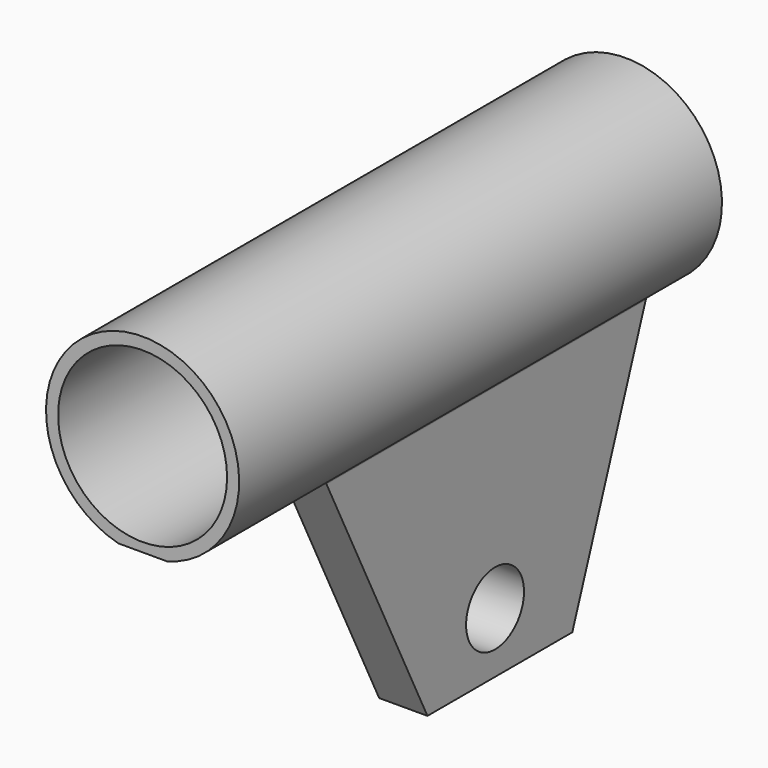
from build123d import *

# Parameters (mm, degrees)
F0_R     = 7
F1_DEPTH = 50
F3_R     = 3
F4_DEPTH = 25
F5_R     = 1.5


with BuildPart() as f1:
    # F0 (on Front) → F1 (new body)
    with BuildSketch(Plane.XZ):
        with BuildLine():
            Line((2, -30), (2, -7.7459666924))
            ThreePointArc((2, -7.7459666924), (0, 8), (-2, -7.7459666924))
            Line((-2, -7.7459666924), (-2, -30))
            Line((-2, -30), (0, -30))
            Line((0, -30), (2, -30))
        make_face()
        Circle(F0_R, mode=Mode.SUBTRACT)
    extrude(amount=F1_DEPTH)

    # F3 (on face) → F4 (cut)
    with BuildSketch(Plane(origin=(-2, 0, 0), x_dir=(0, -1, 0), z_dir=(-1, 0, 0))):
        Polygon((50, -7.7459666924), (34, -7.7459666924), (23, -30), (50, -30), align=None)
        Polygon((8, -30), (0, -7.7459666924), (0, -30), align=None)
        with Locations((16, -25)):
            Circle(F3_R)
    extrude(amount=-F4_DEPTH, mode=Mode.SUBTRACT)

    # F5 (call 1 of 2: OpenCascade refuses the feature's edges together)
    f5_edges = [f1.edges().sort_by_distance(p)[0] for p in [
        (-2, -17, -7.745967),
    ]]
    fillet(f5_edges, radius=F5_R)

    # F5#2 (call 2 of 2)
    f5_2_edges = [f1.edges().sort_by_distance(p)[0] for p in [
        (2, -17, -7.745967),
    ]]
    fillet(f5_2_edges, radius=F5_R)


solid = f1.part
